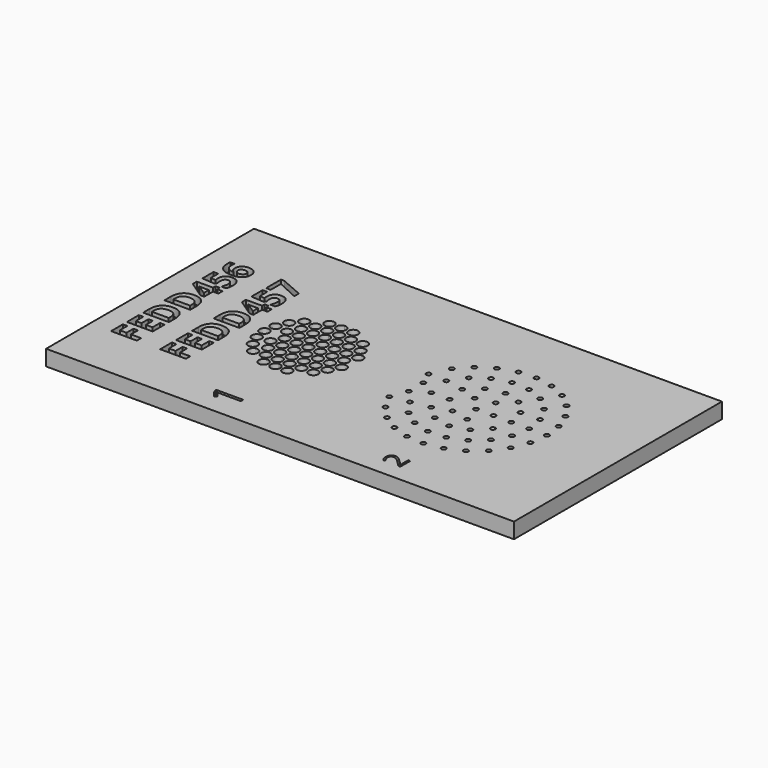
from build123d import *

# Parameters (mm, degrees)
F0_W           = 90
F0_H           = 50
F1_DEPTH       = 3
F2_TEXT_SIZE   = 6.9444444444
F2_TEXT_SIZE_2 = 7.24801812
F2_TEXT_SIZE_3 = 5.1460734388
F3_DEPTH       = 1.5
F4_R           = 0.935
F4_R_2         = 0.45
F5_DEPTH       = 3


# Not quite as in the source:
# - Text() gives the source's letters only with a copy of the font that has no kerning and outlines rounded to 1/6400 em; it was checked with that copy


with BuildPart() as f1:
    # F0 (on Top) → F1 (new body)
    with BuildSketch(Plane.XY):
        with Locations((1.8412768841, 3.3350909071)):
            Rectangle(F0_W, F0_H)
    extrude(amount=F1_DEPTH)

    # F2 (on face) → F3 (cut)
    with BuildSketch(Plane.XY.offset(3)):
        with Locations(Location((-34.1587231159, -11.7149090929), (0, 0, 90))):
            Text('FEDD456', F2_TEXT_SIZE, font='Open Sans', font_style=FontStyle.BOLD, text_align=(TextAlign.LEFT, TextAlign.BOTTOM))
        with Locations(Location((-24.7142786715, -11.7149090929), (0, 0, 90))):
            Text('FEDD457', F2_TEXT_SIZE, font='Open Sans', font_style=FontStyle.BOLD, text_align=(TextAlign.LEFT, TextAlign.BOTTOM))
        with Locations(Location((-9.6570708402, -18.6649090929), (0, 0, 90))):
            Text('1', F2_TEXT_SIZE_2, font='Open Sans', text_align=(TextAlign.LEFT, TextAlign.BOTTOM))
        with Locations(Location((22.3617675547, -18.6649090929), (0, 0, 90))):
            Text('2', F2_TEXT_SIZE_3, font='Open Sans', text_align=(TextAlign.LEFT, TextAlign.BOTTOM))
    extrude(amount=-F3_DEPTH, mode=Mode.SUBTRACT)

    # F4 (on face) → F5 (cut, through all)
    with BuildSketch(Plane.XY.offset(3)):
        with BuildLine():
            ThreePointArc((-20.2237231159, 3.3350909071), (-21.1587231159, 4.2700909071), (-22.0937231159, 3.3350909071))
            Line((-22.0937231159, 3.3350909071), (-20.2237231159, 3.3350909071))
        make_face()
        with BuildLine():
            ThreePointArc((-12.7987231159, 12.184727933), (-13.6337231159, 11.2550909071), (-12.7987231159, 10.3254538811))
            Line((-12.7987231159, 10.3254538811), (-12.7987231159, 12.184727933))
        make_face()
        with BuildLine():
            Line((-12.7987231159, 12.184727933), (-12.7987231159, 10.3254538811))
            ThreePointArc((-12.7987231159, 10.3254538811), (-12.0739331512, 10.55948865), (-11.7637231159, 11.2550909071))
            ThreePointArc((-11.7637231159, 11.2550909071), (-12.0739331512, 11.9506931641), (-12.7987231159, 12.184727933))
        make_face()
        with BuildLine():
            ThreePointArc((-12.7987231159, 8.244727933), (-13.6337231159, 7.3150909071), (-12.7987231159, 6.3854538811))
            Line((-12.7987231159, 6.3854538811), (-12.7987231159, 8.244727933))
        make_face()
        with BuildLine():
            Line((-12.7987231159, 8.244727933), (-12.7987231159, 6.3854538811))
            ThreePointArc((-12.7987231159, 6.3854538811), (-12.0739331512, 6.61948865), (-11.7637231159, 7.3150909071))
            ThreePointArc((-11.7637231159, 7.3150909071), (-12.0739331512, 8.0106931641), (-12.7987231159, 8.244727933))
        make_face()
        with BuildLine():
            ThreePointArc((-4.9037231159, 3.3350909071), (-5.8387231159, 4.2700909071), (-6.7737231159, 3.3350909071))
            Line((-6.7737231159, 3.3350909071), (-4.9037231159, 3.3350909071))
        make_face()
        with BuildLine():
            Line((-4.9037231159, 3.3350909071), (-6.7737231159, 3.3350909071))
            ThreePointArc((-6.7737231159, 3.3350909071), (-5.8387231159, 2.4000909071), (-4.9037231159, 3.3350909071))
        make_face()
        with BuildLine():
            ThreePointArc((-7.1937231159, 3.3350909071), (-8.1287231159, 4.2700909071), (-9.0637231159, 3.3350909071))
            Line((-9.0637231159, 3.3350909071), (-7.1937231159, 3.3350909071))
        make_face()
        with BuildLine():
            Line((-7.1937231159, 3.3350909071), (-9.0637231159, 3.3350909071))
            ThreePointArc((-9.0637231159, 3.3350909071), (-8.1287231159, 2.4000909071), (-7.1937231159, 3.3350909071))
        make_face()
        with BuildLine():
            ThreePointArc((-9.4737231159, 3.3350909071), (-10.4087231159, 4.2700909071), (-11.3437231159, 3.3350909071))
            Line((-11.3437231159, 3.3350909071), (-9.4737231159, 3.3350909071))
        make_face()
        with BuildLine():
            Line((-9.4737231159, 3.3350909071), (-11.3437231159, 3.3350909071))
            ThreePointArc((-11.3437231159, 3.3350909071), (-10.4087231159, 2.4000909071), (-9.4737231159, 3.3350909071))
        make_face()
        with BuildLine():
            ThreePointArc((-11.7637231159, -4.5849090929), (-12.0739331512, -3.8893068359), (-12.7987231159, -3.655272067))
            Line((-12.7987231159, -3.655272067), (-12.7987231159, -5.5145461189))
            ThreePointArc((-12.7987231159, -5.5145461189), (-12.0739331512, -5.28051135), (-11.7637231159, -4.5849090929))
        make_face()
        with BuildLine():
            Line((-12.7987231159, -5.5145461189), (-12.7987231159, -3.655272067))
            ThreePointArc((-12.7987231159, -3.655272067), (-13.6337231159, -4.5849090929), (-12.7987231159, -5.5145461189))
        make_face()
        with BuildLine():
            ThreePointArc((-11.7637231159, -0.6449090929), (-12.0739331512, 0.0506931641), (-12.7987231159, 0.284727933))
            Line((-12.7987231159, 0.284727933), (-12.7987231159, -1.5745461189))
            ThreePointArc((-12.7987231159, -1.5745461189), (-12.0739331512, -1.34051135), (-11.7637231159, -0.6449090929))
        make_face()
        with BuildLine():
            Line((-12.7987231159, -1.5745461189), (-12.7987231159, 0.284727933))
            ThreePointArc((-12.7987231159, 0.284727933), (-13.6337231159, -0.6449090929), (-12.7987231159, -1.5745461189))
        make_face()
        with BuildLine():
            ThreePointArc((-12.7987231159, 4.264727933), (-13.394325373, 3.9598808718), (-13.6337231159, 3.3350909071))
            Line((-13.6337231159, 3.3350909071), (-12.7987231159, 3.3350909071))
            Line((-12.7987231159, 3.3350909071), (-12.7987231159, 4.264727933))
        make_face()
        with BuildLine():
            Line((-12.7987231159, 3.3350909071), (-13.6337231159, 3.3350909071))
            ThreePointArc((-13.6337231159, 3.3350909071), (-13.394325373, 2.7103009423), (-12.7987231159, 2.4054538811))
            Line((-12.7987231159, 2.4054538811), (-12.7987231159, 3.3350909071))
        make_face()
        with BuildLine():
            ThreePointArc((-14.0437231159, 3.3350909071), (-14.9787231159, 4.2700909071), (-15.9137231159, 3.3350909071))
            Line((-15.9137231159, 3.3350909071), (-14.0437231159, 3.3350909071))
        make_face()
        with BuildLine():
            Line((-14.0437231159, 3.3350909071), (-15.9137231159, 3.3350909071))
            ThreePointArc((-15.9137231159, 3.3350909071), (-14.9787231159, 2.4000909071), (-14.0437231159, 3.3350909071))
        make_face()
        with BuildLine():
            ThreePointArc((-16.3337231159, 3.3350909071), (-17.2687231159, 4.2700909071), (-18.2037231159, 3.3350909071))
            Line((-18.2037231159, 3.3350909071), (-16.3337231159, 3.3350909071))
        make_face()
        with BuildLine():
            Line((-16.3337231159, 3.3350909071), (-18.2037231159, 3.3350909071))
            ThreePointArc((-18.2037231159, 3.3350909071), (-17.2687231159, 2.4000909071), (-16.3337231159, 3.3350909071))
        make_face()
        with BuildLine():
            Line((-20.2237231159, 3.3350909071), (-22.0937231159, 3.3350909071))
            ThreePointArc((-22.0937231159, 3.3350909071), (-21.1587231159, 2.4000909071), (-20.2237231159, 3.3350909071))
        make_face()
        with BuildLine():
            Line((-12.7987231159, 4.264727933), (-12.7987231159, 3.3350909071))
            Line((-12.7987231159, 3.3350909071), (-11.7637231159, 3.3350909071))
            ThreePointArc((-11.7637231159, 3.3350909071), (-12.0739331512, 4.0306931641), (-12.7987231159, 4.264727933))
        make_face()
        with BuildLine():
            Line((-11.7637231159, 3.3350909071), (-12.7987231159, 3.3350909071))
            Line((-12.7987231159, 3.3350909071), (-12.7987231159, 2.4054538811))
            ThreePointArc((-12.7987231159, 2.4054538811), (-12.0739331512, 2.63948865), (-11.7637231159, 3.3350909071))
        make_face()
        with Locations((-14.9787231159, -4.5849090929)):
            Circle(F4_R)
        with Locations((-18.4087231159, -2.8149090929)):
            Circle(F4_R)
        with Locations((-19.8887231159, -1.0349090929)):
            Circle(F4_R)
        with Locations((-20.8287231159, 1.0750909071)):
            Circle(F4_R)
        with Locations((-20.8287231159, 5.5950909071)):
            Circle(F4_R)
        with Locations((-19.8887231159, 7.7050909071)):
            Circle(F4_R)
        with Locations((-18.4087231159, 9.4850909071)):
            Circle(F4_R)
        with Locations((-14.9787231159, 11.2550909071)):
            Circle(F4_R)
        with Locations((-10.4087231159, 11.2550909071)):
            Circle(F4_R)
        with Locations((-6.9787231159, 9.2750909071)):
            Circle(F4_R)
        with Locations((-5.8387231159, 7.2950909071)):
            Circle(F4_R)
        with Locations((-4.6987231159, 5.3150909071)):
            Circle(F4_R)
        with Locations((-4.6987231159, 1.3550909071)):
            Circle(F4_R)
        with Locations((-5.8387231159, -0.6249090929)):
            Circle(F4_R)
        with Locations((-6.9787231159, -2.6049090929)):
            Circle(F4_R)
        with Locations((-10.4087231159, -4.5849090929)):
            Circle(F4_R)
        with Locations((-18.4087231159, 5.3150909071)):
            Circle(F4_R)
        with Locations((-17.2687231159, 7.2950909071)):
            Circle(F4_R)
        with Locations((-16.1287231159, 9.2750909071)):
            Circle(F4_R)
        with Locations((-13.8387231159, 9.2750909071)):
            Circle(F4_R)
        with Locations((-16.1287231159, 5.3150909071)):
            Circle(F4_R)
        with Locations((-14.9787231159, 7.2950909071)):
            Circle(F4_R)
        with Locations((-13.8387231159, 5.3150909071)):
            Circle(F4_R)
        with Locations((-9.2687231159, 9.2750909071)):
            Circle(F4_R)
        with Locations((-8.1287231159, 7.2950909071)):
            Circle(F4_R)
        with Locations((-9.2687231159, 5.3150909071)):
            Circle(F4_R)
        with Locations((-10.4087231159, 7.2950909071)):
            Circle(F4_R)
        with Locations((-11.5587231159, 5.3150909071)):
            Circle(F4_R)
        with Locations((-18.4087231159, 1.3550909071)):
            Circle(F4_R)
        with Locations((-16.1287231159, 1.3550909071)):
            Circle(F4_R)
        with Locations((-13.8387231159, 1.3550909071)):
            Circle(F4_R)
        with Locations((-11.5587231159, 1.3550909071)):
            Circle(F4_R)
        with Locations((-9.2687231159, 1.3550909071)):
            Circle(F4_R)
        with Locations((-6.9787231159, 1.3550909071)):
            Circle(F4_R)
        with Locations((-17.2687231159, -0.6249090929)):
            Circle(F4_R)
        with Locations((-14.9787231159, -0.6249090929)):
            Circle(F4_R)
        with Locations((-10.4087231159, -0.6249090929)):
            Circle(F4_R)
        with Locations((-8.1287231159, -0.6249090929)):
            Circle(F4_R)
        with Locations((-16.1287231159, -2.6049090929)):
            Circle(F4_R)
        with Locations((-13.8387231159, -2.6049090929)):
            Circle(F4_R)
        with Locations((-11.5587231159, -2.6049090929)):
            Circle(F4_R)
        with Locations((-9.2687231159, -2.6049090929)):
            Circle(F4_R)
        with Locations((-6.9787231159, 5.3150909071)):
            Circle(F4_R)
        with Locations((-11.5587231159, 9.2750909071)):
            Circle(F4_R)
        with BuildLine():
            ThreePointArc((11.4012768841, 3.3350909071), (10.9512768841, 3.7850909071), (10.5012768841, 3.3350909071))
            Line((10.5012768841, 3.3350909071), (11.4012768841, 3.3350909071))
        make_face()
        with BuildLine():
            ThreePointArc((19.5412768841, 10.4892566457), (19.3412768841, 10.1150909071), (19.5412768841, 9.7409251684))
            Line((19.5412768841, 9.7409251684), (19.5412768841, 10.4892566457))
        make_face()
        with BuildLine():
            Line((19.5412768841, 10.4892566457), (19.5412768841, 9.7409251684))
            ThreePointArc((19.5412768841, 9.7409251684), (20.0034089184, 9.7182282104), (20.2412768841, 10.1150909071))
            ThreePointArc((20.2412768841, 10.1150909071), (20.0034089184, 10.5119536037), (19.5412768841, 10.4892566457))
        make_face()
        with BuildLine():
            ThreePointArc((33.6312768841, 3.3350909071), (33.1812768841, 3.7850909071), (32.7312768841, 3.3350909071))
            Line((32.7312768841, 3.3350909071), (33.6312768841, 3.3350909071))
        make_face()
        with BuildLine():
            Line((33.6312768841, 3.3350909071), (32.7312768841, 3.3350909071))
            ThreePointArc((32.7312768841, 3.3350909071), (33.1812768841, 2.8850909071), (33.6312768841, 3.3350909071))
        make_face()
        with BuildLine():
            ThreePointArc((30.2012768841, 3.3350909071), (29.7512768841, 3.7850909071), (29.3012768841, 3.3350909071))
            Line((29.3012768841, 3.3350909071), (30.2012768841, 3.3350909071))
        make_face()
        with BuildLine():
            Line((30.2012768841, 3.3350909071), (29.3012768841, 3.3350909071))
            ThreePointArc((29.3012768841, 3.3350909071), (29.7512768841, 2.8850909071), (30.2012768841, 3.3350909071))
        make_face()
        with BuildLine():
            ThreePointArc((26.7712768841, 3.3350909071), (26.3212768841, 3.7850909071), (25.8712768841, 3.3350909071))
            Line((25.8712768841, 3.3350909071), (26.7712768841, 3.3350909071))
        make_face()
        with BuildLine():
            Line((26.7712768841, 3.3350909071), (25.8712768841, 3.3350909071))
            ThreePointArc((25.8712768841, 3.3350909071), (26.3212768841, 2.8850909071), (26.7712768841, 3.3350909071))
        make_face()
        with BuildLine():
            ThreePointArc((23.3412768841, 3.3350909071), (22.8912768841, 3.7850909071), (22.4412768841, 3.3350909071))
            Line((22.4412768841, 3.3350909071), (23.3412768841, 3.3350909071))
        make_face()
        with BuildLine():
            Line((23.3412768841, 3.3350909071), (22.4412768841, 3.3350909071))
            ThreePointArc((22.4412768841, 3.3350909071), (22.8912768841, 2.8850909071), (23.3412768841, 3.3350909071))
        make_face()
        with BuildLine():
            ThreePointArc((20.2412768841, -3.4449090929), (20.0034089184, -3.0480463963), (19.5412768841, -3.0707433543))
            Line((19.5412768841, -3.0707433543), (19.5412768841, -3.8190748316))
            ThreePointArc((19.5412768841, -3.8190748316), (20.0034089184, -3.8417717896), (20.2412768841, -3.4449090929))
        make_face()
        with BuildLine():
            Line((19.5412768841, -3.8190748316), (19.5412768841, -3.0707433543))
            ThreePointArc((19.5412768841, -3.0707433543), (19.3412768841, -3.4449090929), (19.5412768841, -3.8190748316))
        make_face()
        with BuildLine():
            ThreePointArc((19.5412768841, 3.7850909071), (19.2230788325, 3.6532889586), (19.0912768841, 3.3350909071))
            Line((19.0912768841, 3.3350909071), (19.5412768841, 3.3350909071))
            Line((19.5412768841, 3.3350909071), (19.5412768841, 3.7850909071))
        make_face()
        with BuildLine():
            Line((19.5412768841, 3.3350909071), (19.0912768841, 3.3350909071))
            ThreePointArc((19.0912768841, 3.3350909071), (19.2230788325, 3.0168928555), (19.5412768841, 2.8850909071))
            Line((19.5412768841, 2.8850909071), (19.5412768841, 3.3350909071))
        make_face()
        with BuildLine():
            ThreePointArc((14.9112768841, 3.3350909071), (14.4612768841, 3.7850909071), (14.0112768841, 3.3350909071))
            Line((14.0112768841, 3.3350909071), (14.9112768841, 3.3350909071))
        make_face()
        with BuildLine():
            Line((14.9112768841, 3.3350909071), (14.0112768841, 3.3350909071))
            ThreePointArc((14.0112768841, 3.3350909071), (14.4612768841, 2.8850909071), (14.9112768841, 3.3350909071))
        make_face()
        with BuildLine():
            Line((11.4012768841, 3.3350909071), (10.5012768841, 3.3350909071))
            ThreePointArc((10.5012768841, 3.3350909071), (10.9512768841, 2.8850909071), (11.4012768841, 3.3350909071))
        make_face()
        with BuildLine():
            Line((19.5412768841, 3.7850909071), (19.5412768841, 3.3350909071))
            Line((19.5412768841, 3.3350909071), (19.9912768841, 3.3350909071))
            ThreePointArc((19.9912768841, 3.3350909071), (19.8594749356, 3.6532889586), (19.5412768841, 3.7850909071))
        make_face()
        with BuildLine():
            Line((19.9912768841, 3.3350909071), (19.5412768841, 3.3350909071))
            Line((19.5412768841, 3.3350909071), (19.5412768841, 2.8850909071))
            ThreePointArc((19.5412768841, 2.8850909071), (19.8594749356, 3.0168928555), (19.9912768841, 3.3350909071))
        make_face()
        with Locations((6.8412768841, 7.8150909071)):
            Circle(F4_R_2)
        with Locations((8.4912768841, 11.3150909071)):
            Circle(F4_R_2)
        with Locations((10.8312768841, 13.8250909071)):
            Circle(F4_R_2)
        with Locations((13.7012768841, 15.6550909071)):
            Circle(F4_R_2)
        with Locations((16.9712768841, 16.7250909071)):
            Circle(F4_R_2)
        with Locations((20.3012768841, 16.9450909071)):
            Circle(F4_R_2)
        with Locations((23.7112768841, 16.3150909071)):
            Circle(F4_R_2)
        with Locations((26.8312768841, 14.8650909071)):
            Circle(F4_R_2)
        with Locations((29.4712768841, 12.6850909071)):
            Circle(F4_R_2)
        with Locations((31.4812768841, 9.9150909071)):
            Circle(F4_R_2)
        with Locations((32.7212768841, 6.7350909071)):
            Circle(F4_R_2)
        with Locations((32.7212768841, -0.0649090929)):
            Circle(F4_R_2)
        with Locations((31.4812768841, -3.2449090929)):
            Circle(F4_R_2)
        with Locations((29.4712768841, -6.0149090929)):
            Circle(F4_R_2)
        with Locations((26.8312768841, -8.1949090929)):
            Circle(F4_R_2)
        with Locations((23.7112768841, -9.6449090929)):
            Circle(F4_R_2)
        with Locations((20.3012768841, -10.2749090929)):
            Circle(F4_R_2)
        with Locations((16.9712768841, -10.0549090929)):
            Circle(F4_R_2)
        with Locations((13.7012768841, -8.9849090929)):
            Circle(F4_R_2)
        with Locations((10.8312768841, -7.1549090929)):
            Circle(F4_R_2)
        with Locations((8.4912768841, -4.6449090929)):
            Circle(F4_R_2)
        with Locations((6.8412768841, -1.6449090929)):
            Circle(F4_R_2)
        with Locations((8.0112768841, 5.0650909071)):
            Circle(F4_R_2)
        with Locations((10.3212768841, 7.7250909071)):
            Circle(F4_R_2)
        with Locations((12.3512768841, 10.5750909071)):
            Circle(F4_R_2)
        with Locations((15.0912768841, 12.5250909071)):
            Circle(F4_R_2)
        with Locations((18.3712768841, 13.4650909071)):
            Circle(F4_R_2)
        with Locations((21.7812768841, 13.2950909071)):
            Circle(F4_R_2)
        with Locations((24.9512768841, 11.9950909071)):
            Circle(F4_R_2)
        with Locations((27.5212768841, 9.7150909071)):
            Circle(F4_R_2)
        with Locations((23.0712768841, 9.1250909071)):
            Circle(F4_R_2)
        with Locations((25.4612768841, 6.6650909071)):
            Circle(F4_R_2)
        with Locations((20.5812768841, 6.7650909071)):
            Circle(F4_R_2)
        with Locations((13.8812768841, 7.0650909071)):
            Circle(F4_R_2)
        with Locations((16.4412768841, 9.3550909071)):
            Circle(F4_R_2)
        with Locations((17.1512768841, 6.0050909071)):
            Circle(F4_R_2)
        with Locations((8.0112768841, 1.6050909071)):
            Circle(F4_R_2)
        with Locations((10.3212768841, -1.0549090929)):
            Circle(F4_R_2)
        with Locations((12.3512768841, -3.9049090929)):
            Circle(F4_R_2)
        with Locations((15.0912768841, -5.8549090929)):
            Circle(F4_R_2)
        with Locations((18.3712768841, -6.7949090929)):
            Circle(F4_R_2)
        with Locations((13.8812768841, -0.3949090929)):
            Circle(F4_R_2)
        with Locations((16.4412768841, -2.6849090929)):
            Circle(F4_R_2)
        with Locations((17.1512768841, 0.6650909071)):
            Circle(F4_R_2)
        with Locations((25.4612768841, 0.0050909071)):
            Circle(F4_R_2)
        with Locations((29.1712768841, -0.0449090929)):
            Circle(F4_R_2)
        with Locations((27.5212768841, -3.0449090929)):
            Circle(F4_R_2)
        with Locations((24.9512768841, -5.3149090929)):
            Circle(F4_R_2)
        with Locations((21.7812768841, -6.6249090929)):
            Circle(F4_R_2)
        with Locations((20.5812768841, -0.0949090929)):
            Circle(F4_R_2)
        with Locations((29.1712768841, 6.7150909071)):
            Circle(F4_R_2)
        with Locations((23.0712768841, -2.4549090929)):
            Circle(F4_R_2)
    extrude(amount=-F5_DEPTH, mode=Mode.SUBTRACT)


solid = f1.part
